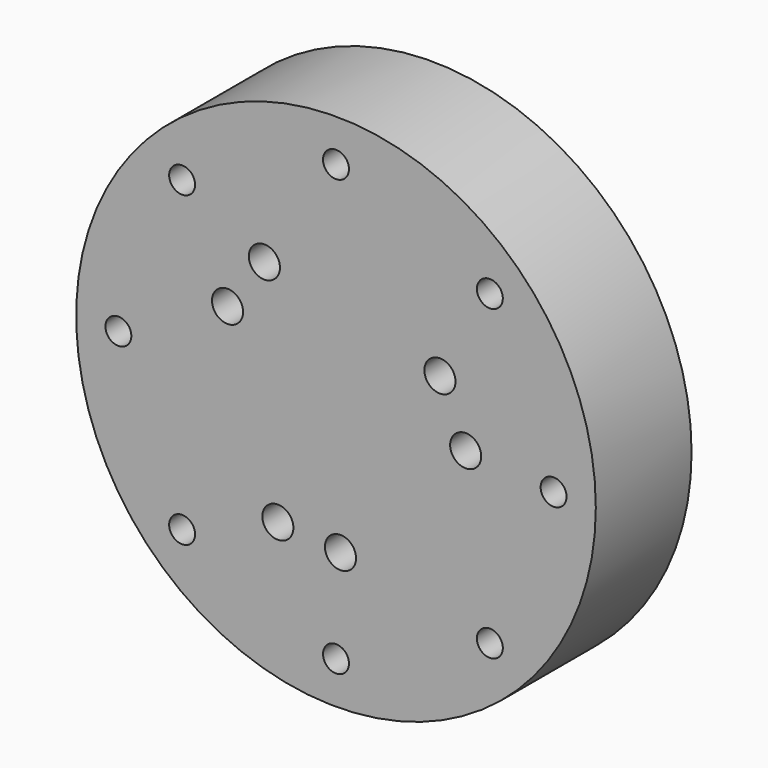
from build123d import *

# Parameters (mm, degrees)
F0_R           = 55.1311075469
F2_DEPTH       = 25.4
F3_D           = 5.5
F3_CBORE_D     = 9.75
F3_CBORE_DEPTH = 5
F4_D           = 6.6
F4_CBORE_D     = 11.25
F4_CBORE_DEPTH = 6


with BuildPart() as f2:
    # F0 (on Front) → F2 (new body)
    with BuildSketch(Plane.XZ):
        Circle(F0_R)
    extrude(amount=F2_DEPTH)

    # F3 (through all)
    with Locations(Plane(origin=(0, 0, 0), x_dir=(1, 0, 0), z_dir=(0, 1, 0))):
        with Locations((-32.6479577467, -32.6479577467), (0, -46.1711846292), (32.6479577467, -32.6479577467), (46.1711846292, 0), (32.6479577467, 32.6479577467), (0, 46.1711846292), (-46.1711846292, 0), (-32.6479577467, 32.6479577467)):
            CounterBoreHole(F3_D / 2, F3_CBORE_D / 2, F3_CBORE_DEPTH)

    # F4 (through all)
    with Locations(Plane(origin=(0, 0, 0), x_dir=(1, 0, 0), z_dir=(0, 1, 0))):
        with Locations((-12.3326523611, 24.660010453), (0.9552987674, 26.0185740339), (-23.0103954673, -12.1819740161), (-15.1898693293, -23.0103954673), (22.0550966999, -13.8366000177), (27.5225216905, -1.6496149857)):
            CounterBoreHole(F4_D / 2, F4_CBORE_D / 2, F4_CBORE_DEPTH)


solid = f2.part
